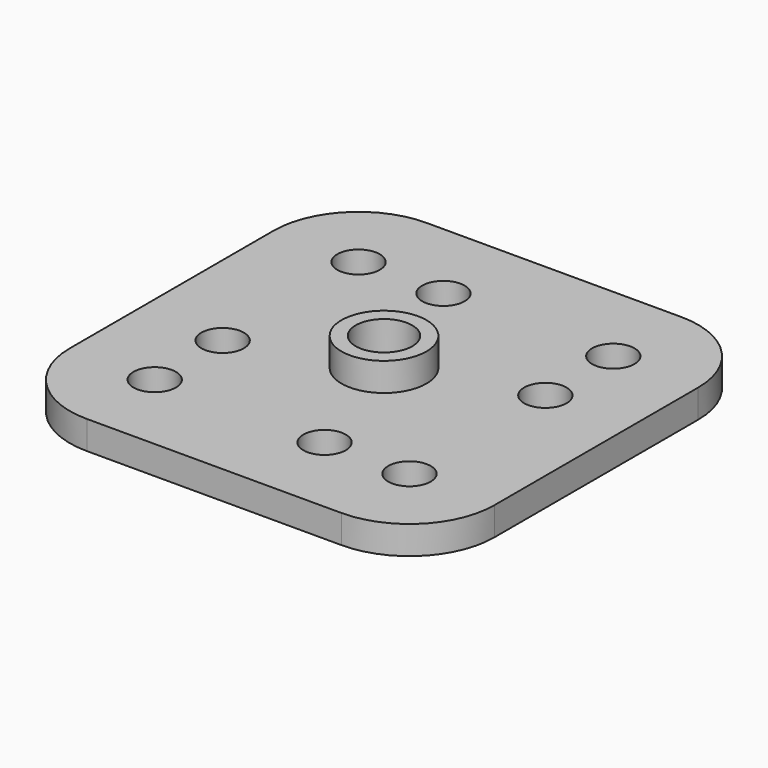
from build123d import *

# Parameters (mm, degrees)
F0_R            = 1.5
F0_R_2          = 1
F1_DEPTH        = 1
F2_W            = 15
F2_H            = 15
F2_R            = 5
F2_R_2          = 1.5
F2_R_3          = 1
F3_DEPTH        = 1
F4_R            = 3
F5_R            = 0.75
F6_DEPTH        = 25
F6_COPIES_COUNT = 4


# Not quite as in the source:
# - a pattern or mirror of a feature is missing from the dataset's text; its kind, count and spacing are read off the source's solid


with BuildPart() as f1:
    # F0 (on Top) → F1 (new body)
    with BuildSketch(Plane.XY):
        Circle(F0_R)
        Circle(F0_R_2, mode=Mode.SUBTRACT)
    extrude(amount=F1_DEPTH)

    # F2 (on face) → F3 (join)
    with BuildSketch(Plane(origin=(0, 0, 0), x_dir=(1, 0, 0), z_dir=(0, 0, -1))):
        Rectangle(F2_W, F2_H)
        Circle(F2_R, mode=Mode.SUBTRACT)
        Circle(F2_R)
        Circle(F2_R_2, mode=Mode.SUBTRACT)
        Circle(F2_R_2)
        Circle(F2_R_3, mode=Mode.SUBTRACT)
    extrude(amount=F3_DEPTH)

    # F4
    f4_edges = [f1.edges().sort_by_distance(p)[0] for p in [
        (-7.5, 7.5, -0.5),
        (7.5, 7.5, -0.5),
        (-7.5, -7.5, -0.5),
        (7.5, -7.5, -0.5),
    ]]
    fillet(f4_edges, radius=F4_R)

    # F5 (on face) → F6 (cut)
    with BuildSketch(Plane.XY):
        with Locations((-4.5, 4.5)):
            Circle(F5_R)
        with Locations((-1.5, 4.5)):
            Circle(F5_R)
    f6 = extrude(amount=-F6_DEPTH, mode=Mode.SUBTRACT)

    # F6_copies: F6 ×4 about axis
    f6_copies_axis = Axis((0, 0, 0), (0, 0, 1))
    for i in range(1, F6_COPIES_COUNT):
        add(f6.rotate(f6_copies_axis, i * 360 / F6_COPIES_COUNT), mode=Mode.SUBTRACT)


solid = f1.part
